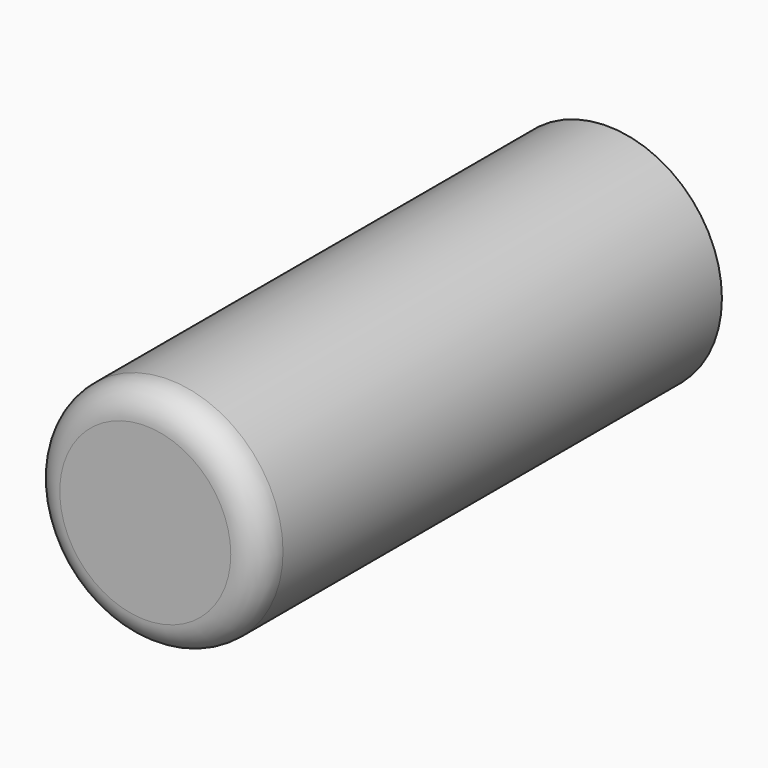
from build123d import *

# Parameters (mm, degrees)
F0_R     = 10.0216829106
F1_DEPTH = 50.546
F2_R     = 2.54


# Not quite as in the source:
# - the program builds the solid bodies; features that only make, move or delete a surface that nothing else refers to are left out


with BuildPart() as f1:
    # F0 (on Front) → F1 (new body)
    with BuildSketch(Plane.XZ):
        with Locations((-54.8081733286, 35.9677970409)):
            Circle(F0_R)
    extrude(amount=F1_DEPTH)

    # F2
    f2_edges = [f1.edges().sort_by_distance(p)[0] for p in [
        (-64.829856, -50.546, 35.967797),
    ]]
    fillet(f2_edges, radius=F2_R)


solid = f1.part
